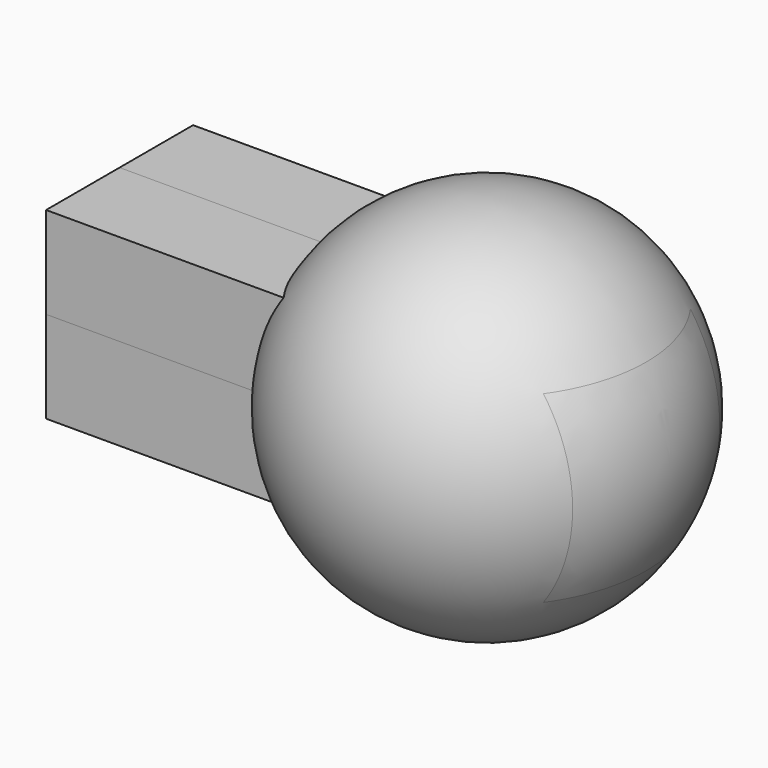
from build123d import *

# Parameters (mm, degrees)
F2_W     = 25
F2_H     = 25
F3_REACH = 110.3563390593


with BuildPart() as f1:
    # F0 (on Front) → F1 (revolve)
    with BuildSketch(Plane.XZ):
        with BuildLine():
            Line((0, 12.5), (0, 0))
            Line((0, 0), (25, 0))
            Line((25, 0), (50, 0))
            Line((50, 0), (75, 0))
            ThreePointArc((75, 0), (56.4704761276, 24.1481456572), (28.3493649054, 12.5))
            Line((28.3493649054, 12.5), (0, 12.5))
        make_face()
    revolve(axis=Axis((12.5, 0, 0), (1, 0, 0)))

    f3_end = f1.faces().sort_by_distance((56.4704761276, 0, -24.1481456572))[0]
    # F2 (on face) → F3 (join, up to a face of the model that its end follows)
    with BuildSketch(Plane(origin=(0, 0, 0), x_dir=(0, -1, 0), z_dir=(-1, 0, 0))):
        Rectangle(F2_W, F2_H)
    f3_long = extrude(amount=-F3_REACH, mode=Mode.PRIVATE)
    add(split(f3_long, bisect_by=f3_end, keep=Keep.ALL, mode=Mode.PRIVATE).solids().sort_by_distance((0, 0, 0))[0])


solid = f1.part
